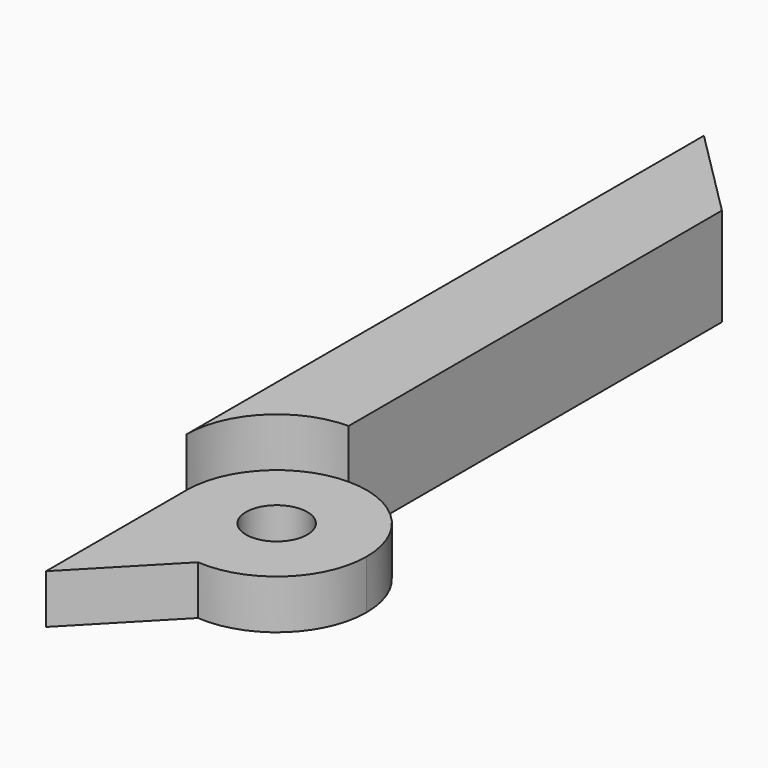
from build123d import *

# Parameters (mm, degrees)
F1_DEPTH    = 7.62
F3_DEPTH    = 3.81
F5_DEPTH    = 3.81
F7_D        = 4.7625
F7_DEPTH    = 12.7
F7_TIP      = 1.4307993491
F8_T1_DEPTH = 46.8124487366


# Not quite as in the source:
# - a fillet or chamfer that OpenCascade refuses, or shapes differently, is made with other operations: its cross-section is extruded or revolved along the edge and cut away or added


with BuildPart() as f1:
    # F0 (on Top) → F1 (new body)
    with BuildSketch(Plane.XY):
        with BuildLine():
            Line((6.985, 27.4185502146), (0, 27.4185502146))
            Line((0, 27.4185502146), (0, -23.3814497854))
            ThreePointArc((0, -23.3814497854), (2.0458591334, -18.4423089188), (6.985, -16.3964497854))
            Line((6.985, -16.3964497854), (6.985, 27.4185502146))
        make_face()
        with BuildLine():
            ThreePointArc((6.985, -16.3964497854), (2.0458591334, -18.4423089188), (0, -23.3814497854))
            Line((0, -23.3814497854), (6.985, -23.3814497854))
            Line((6.985, -23.3814497854), (6.985, -16.3964497854))
        make_face()
        with BuildLine():
            Line((6.985, -23.3814497854), (0, -23.3814497854))
            ThreePointArc((0, -23.3814497854), (6.985, -30.3664497854), (13.97, -23.3814497854))
            ThreePointArc((13.97, -23.3814497854), (11.9241408666, -18.4423089188), (6.985, -16.3964497854))
            Line((6.985, -16.3964497854), (6.985, -23.3814497854))
        make_face()
    extrude(amount=F1_DEPTH)

    # F2 (on face) → F3 (cut)
    with BuildSketch(Plane.XY.offset(7.62)):
        with BuildLine():
            ThreePointArc((0, -23.3814497854), (6.985, -30.3664497854), (13.97, -23.3814497854))
            ThreePointArc((13.97, -23.3814497854), (11.9241408666, -18.4423089188), (6.985, -16.3964497854))
            ThreePointArc((6.985, -16.3964497854), (2.0458591334, -18.4423089188), (0, -23.3814497854))
        make_face()
    extrude(amount=-F3_DEPTH, mode=Mode.SUBTRACT)

    # F4 (on face) → F5 (join)
    with BuildSketch(Plane(origin=(0, 0, 0), x_dir=(1, 0, 0), z_dir=(0, 0, -1))):
        with BuildLine():
            Line((0, 37.0080322027), (0, 23.3814497854))
            ThreePointArc((0, 23.3814497854), (1.8603767117, 28.1278653964), (6.4505257418, 30.345971468))
            Line((6.4505257418, 30.345971468), (0, 37.0080322027))
        make_face()
    extrude(amount=-F5_DEPTH)

    # F7
    with Locations(Plane.XY.offset(3.81)):
        with Locations((6.985, -23.3814497854)):
            Hole(F7_D / 2, depth=F7_DEPTH)
            with Locations((0, 0, -(F7_DEPTH + F7_TIP / 2))):  # 118° drill point
                Cone(0, F7_D / 2, F7_TIP, mode=Mode.SUBTRACT)

    # F8: chamfer of 7.62 on 1 edges, made by hand

    # F8_s2 → F8_t1 (cut)
    with BuildSketch(Plane.XY.offset(-19.5962243683)):
        Polygon((-0.635, 27.4185502146), (6.985, 19.7985502146), (6.985, 27.4185502146), align=None)
    extrude(amount=F8_T1_DEPTH, mode=Mode.SUBTRACT)


solid = f1.part
